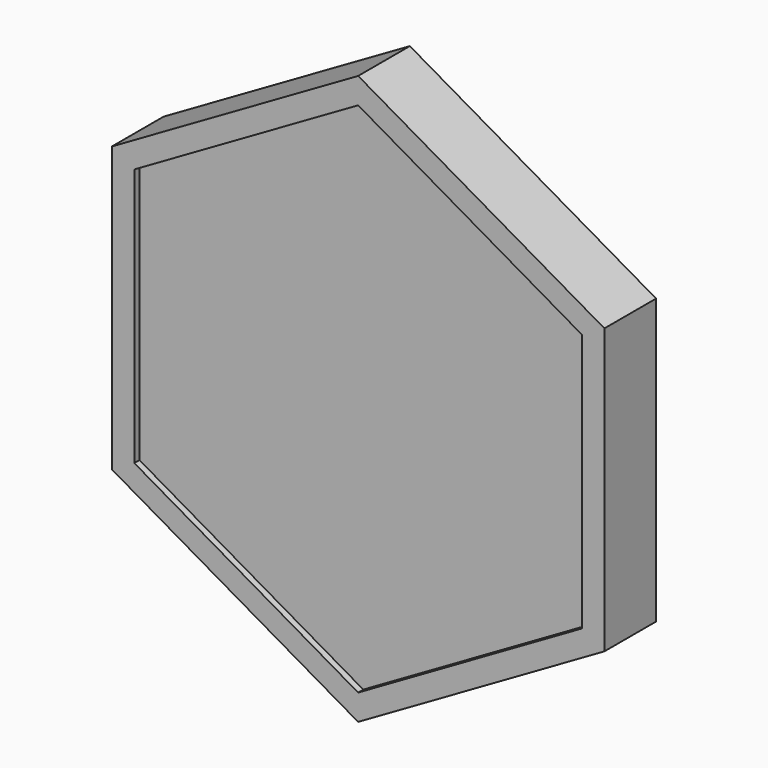
from build123d import *

# Parameters (mm, degrees)
F1_DEPTH = 12.7
F3_DEPTH = 1.27
F4_DEPTH = 11.43


with BuildPart() as f1:
    # F0 (on Front) → F1 (new body)
    with BuildSketch(Plane.XZ):
        Polygon((0.0012905122, 50.7992549224), (-43.9928, 25.3992549224), (-43.9928, -25.4007450776), (-7.57e-08, -50.8029803104), (43.9940904365, -25.4029803104), (43.9940904365, 25.3970196896), align=None)
    extrude(amount=F1_DEPTH)


with BuildPart() as f3:
    # F2 (on face) → F3 (new body)
    with BuildSketch(Plane.XZ.offset(12.7)):
        Polygon((48.3934995635, 27.94), (0, 55.88), (-48.3934995635, 27.94), (-48.3934995635, -27.94), (0, -55.88), (48.3934995635, -27.94), align=None)
        Polygon((-43.9928, -25.4007450776), (-43.9928, 25.3992549224), (0.0012905122, 50.7992549224), (43.9940904365, 25.3970196896), (43.9940904365, -25.4029803104), (-7.57e-08, -50.8029803104), align=None, mode=Mode.SUBTRACT)
    extrude(amount=F3_DEPTH)

    # F4 (add): a face of the model
    f4_faces = [f3.faces().sort_by_distance(p)[0] for p in [
        (46.9150537309, -12.7, 0),
    ]]
    extrude(f4_faces, amount=F4_DEPTH)


solid = Compound([f1.part, f3.part])
